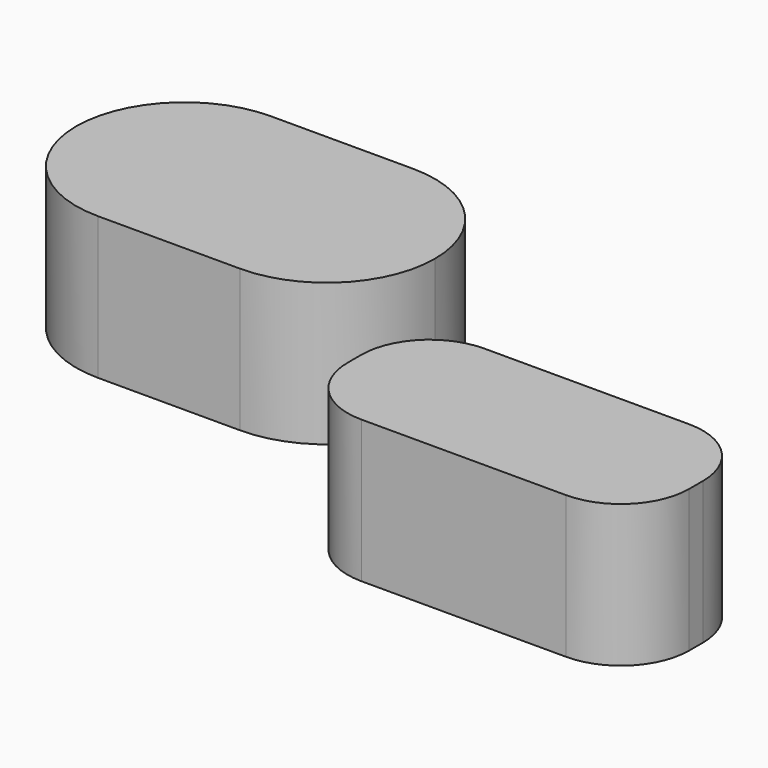
from build123d import *

# Parameters (mm, degrees)
F1_DEPTH = 25
F3_DEPTH = 25


with BuildPart() as f1:
    # F0 (on Top) → F1 (new body)
    with BuildSketch(Plane.XY):
        with BuildLine():
            ThreePointArc((-1.3728568151, 14.3090880213), (-7.1972546851, 17.7886575154), (-13.8728568151, 19))
            ThreePointArc((-13.8728568151, 19), (-32.8728568151, 0), (-13.8728568151, -19))
            ThreePointArc((-13.8728568151, -19), (-7.1972546851, -17.7886575154), (-1.3728568151, -14.3090880213))
            ThreePointArc((-1.3728568151, -14.3090880213), (-7.8728568151, 0), (-1.3728568151, 14.3090880213))
        make_face()
        with BuildLine():
            Line((11.1271431849, 19), (-13.8728568151, 19))
            ThreePointArc((-13.8728568151, 19), (-7.1972546851, 17.7886575154), (-1.3728568151, 14.3090880213))
            ThreePointArc((-1.3728568151, 14.3090880213), (4.4515410549, 17.7886575154), (11.1271431849, 19))
        make_face()
        with BuildLine():
            ThreePointArc((-1.3728568151, -14.3090880213), (-7.1972546851, -17.7886575154), (-13.8728568151, -19))
            Line((-13.8728568151, -19), (11.1271431849, -19))
            ThreePointArc((11.1271431849, -19), (4.4515410549, -17.7886575154), (-1.3728568151, -14.3090880213))
        make_face()
        with BuildLine():
            ThreePointArc((11.1271431849, 19), (4.4515410549, 17.7886575154), (-1.3728568151, 14.3090880213))
            ThreePointArc((-1.3728568151, 14.3090880213), (3.4259870769, 7.8581168228), (5.1271431849, 0))
            ThreePointArc((5.1271431849, 0), (3.4259870769, -7.8581168228), (-1.3728568151, -14.3090880213))
            ThreePointArc((-1.3728568151, -14.3090880213), (4.4515410549, -17.7886575154), (11.1271431849, -19))
            ThreePointArc((11.1271431849, -19), (24.5621720274, -13.4350288425), (30.1271431849, 0))
            ThreePointArc((30.1271431849, 0), (24.5621720274, 13.4350288425), (11.1271431849, 19))
        make_face()
        with BuildLine():
            ThreePointArc((5.1271431849, 0), (3.4259870769, 7.8581168228), (-1.3728568151, 14.3090880213))
            ThreePointArc((-1.3728568151, 14.3090880213), (-7.8728568151, 0), (-1.3728568151, -14.3090880213))
            ThreePointArc((-1.3728568151, -14.3090880213), (3.4259870769, -7.8581168228), (5.1271431849, 0))
        make_face()
    extrude(amount=F1_DEPTH)


with BuildPart() as f3:
    # F2 (on Top) → F3 (new body)
    with BuildSketch(Plane.XY):
        with BuildLine():
            ThreePointArc((40.1626702507, -30.1011827665), (40.0921040397, -30.849707816), (40.0685511505, -31.6011827665))
            ThreePointArc((40.0685511505, -31.6011827665), (43.5832697763, -40.0864641407), (52.0685511505, -43.6011827665))
            ThreePointArc((52.0685511505, -43.6011827665), (60.5538325247, -40.0864641407), (64.0685511505, -31.6011827665))
            ThreePointArc((64.0685511505, -31.6011827665), (64.0449982613, -30.849707816), (63.9744320503, -30.1011827665))
            ThreePointArc((63.9744320503, -30.1011827665), (52.0685511505, -40.6011827665), (40.1626702507, -30.1011827665))
        make_face()
        with BuildLine():
            Line((40.0685511505, -28.6011827665), (40.0685511505, -31.6011827665))
            ThreePointArc((40.0685511505, -31.6011827665), (40.0921040397, -30.849707816), (40.1626702507, -30.1011827665))
            ThreePointArc((40.1626702507, -30.1011827665), (40.0921040397, -29.352657717), (40.0685511505, -28.6011827665))
        make_face()
        with BuildLine():
            ThreePointArc((64.0685511505, -31.6011827665), (60.5538325247, -40.0864641407), (52.0685511505, -43.6011827665))
            Line((52.0685511505, -43.6011827665), (88.0685511505, -43.6011827665))
            ThreePointArc((88.0685511505, -43.6011827665), (79.0685511505, -39.5384366997), (76.1626702507, -30.1011827665))
            ThreePointArc((76.1626702507, -30.1011827665), (79.0685511505, -20.6639288333), (88.0685511505, -16.6011827665))
            Line((88.0685511505, -16.6011827665), (52.0685511505, -16.6011827665))
            ThreePointArc((52.0685511505, -16.6011827665), (60.5538325247, -20.1159013923), (64.0685511505, -28.6011827665))
            ThreePointArc((64.0685511505, -28.6011827665), (64.0449982613, -29.352657717), (63.9744320503, -30.1011827665))
            ThreePointArc((63.9744320503, -30.1011827665), (64.0449982613, -30.849707816), (64.0685511505, -31.6011827665))
        make_face()
        with BuildLine():
            ThreePointArc((40.0685511505, -28.6011827665), (40.0921040397, -29.352657717), (40.1626702507, -30.1011827665))
            ThreePointArc((40.1626702507, -30.1011827665), (52.0685511505, -19.6011827665), (63.9744320503, -30.1011827665))
            ThreePointArc((63.9744320503, -30.1011827665), (64.0449982613, -29.352657717), (64.0685511505, -28.6011827665))
            ThreePointArc((64.0685511505, -28.6011827665), (60.5538325247, -20.1159013923), (52.0685511505, -16.6011827665))
            ThreePointArc((52.0685511505, -16.6011827665), (43.5832697763, -20.1159013923), (40.0685511505, -28.6011827665))
        make_face()
        with BuildLine():
            ThreePointArc((63.9744320503, -30.1011827665), (52.0685511505, -19.6011827665), (40.1626702507, -30.1011827665))
            ThreePointArc((40.1626702507, -30.1011827665), (52.0685511505, -40.6011827665), (63.9744320503, -30.1011827665))
        make_face()
        with BuildLine():
            ThreePointArc((76.1626702507, -30.1011827665), (79.0685511505, -39.5384366997), (88.0685511505, -43.6011827665))
            ThreePointArc((88.0685511505, -43.6011827665), (96.5538325247, -40.0864641407), (100.0685511505, -31.6011827665))
            ThreePointArc((100.0685511505, -31.6011827665), (100.0449982613, -30.849707816), (99.9744320503, -30.1011827665))
            ThreePointArc((99.9744320503, -30.1011827665), (88.0685511505, -40.6011827665), (76.1626702507, -30.1011827665))
        make_face()
        with BuildLine():
            ThreePointArc((99.9744320503, -30.1011827665), (100.0449982613, -30.849707816), (100.0685511505, -31.6011827665))
            Line((100.0685511505, -31.6011827665), (100.0685511505, -28.6011827665))
            ThreePointArc((100.0685511505, -28.6011827665), (100.0449982613, -29.352657717), (99.9744320503, -30.1011827665))
        make_face()
        with BuildLine():
            ThreePointArc((99.9744320503, -30.1011827665), (88.0685511505, -19.6011827665), (76.1626702507, -30.1011827665))
            ThreePointArc((76.1626702507, -30.1011827665), (88.0685511505, -40.6011827665), (99.9744320503, -30.1011827665))
        make_face()
        with BuildLine():
            ThreePointArc((88.0685511505, -16.6011827665), (79.0685511505, -20.6639288333), (76.1626702507, -30.1011827665))
            ThreePointArc((76.1626702507, -30.1011827665), (88.0685511505, -19.6011827665), (99.9744320503, -30.1011827665))
            ThreePointArc((99.9744320503, -30.1011827665), (100.0449982613, -29.352657717), (100.0685511505, -28.6011827665))
            ThreePointArc((100.0685511505, -28.6011827665), (96.5538325247, -20.1159013923), (88.0685511505, -16.6011827665))
        make_face()
    extrude(amount=F3_DEPTH)


solid = Compound([f1.part, f3.part])
